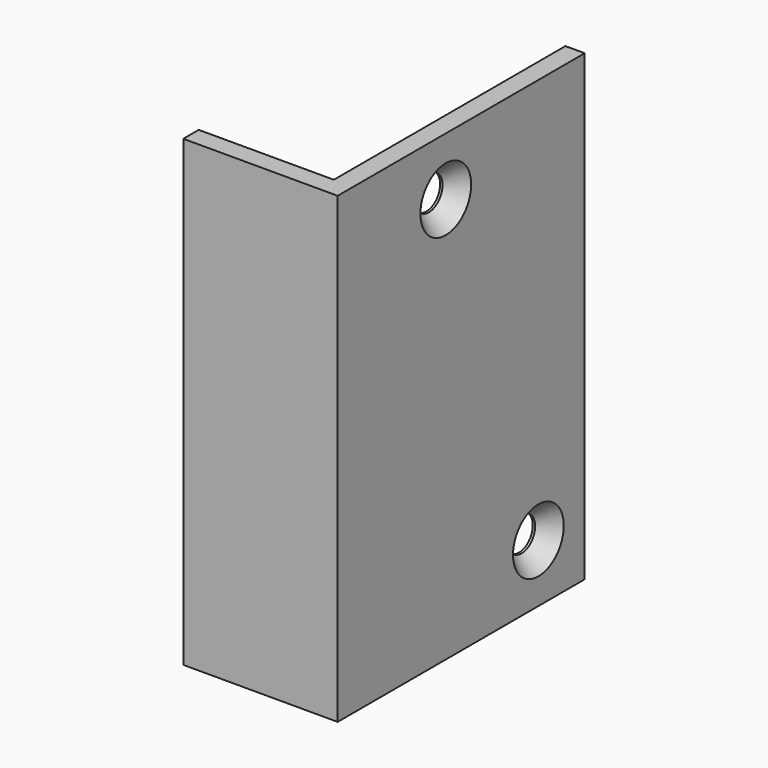
from build123d import *

# Parameters (mm, degrees)
F0_W           = 50.8
F0_H           = 76.2
F1_DEPTH       = 25.4
F3_D           = 5.6134
F3_CSINK_D     = 10.4394
F3_CSINK_ANGLE = 82
F4_W           = 22.225
F4_H           = 47.625
F5_DEPTH       = 76.201


# Not quite as in the source:
# - a feature names something its author has since deleted; it is built from what else it names


with BuildPart() as f1:
    # F0 (on Right) → F1 (new body)
    with BuildSketch(Plane.YZ):
        Rectangle(F0_W, F0_H)
    extrude(amount=F1_DEPTH)

    # F3 (through all)
    with Locations(Plane.YZ.offset(25.4)):
        with Locations((-3.175, 28.575), (15.875, -28.575)):
            CounterSinkHole(F3_D / 2, F3_CSINK_D / 2, counter_sink_angle=F3_CSINK_ANGLE)

    # F4 (on face) → F5 (cut, through all)
    with BuildSketch(Plane.XY.offset(38.1)):
        with Locations((11.1125, 1.5875)):
            Rectangle(F4_W, F4_H)
    extrude(amount=-F5_DEPTH, mode=Mode.SUBTRACT)


solid = f1.part
